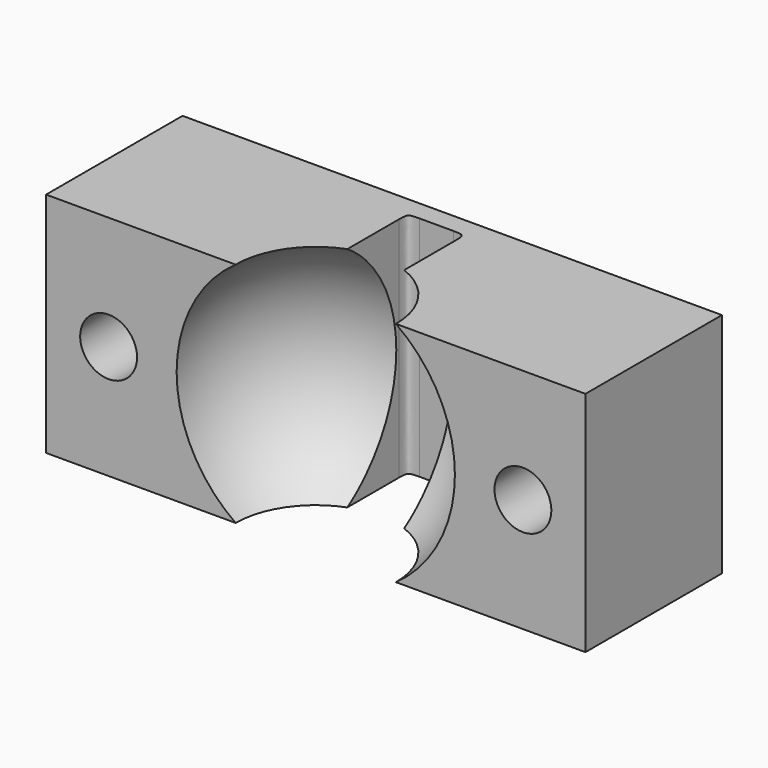
from build123d import *

# Parameters (mm, degrees)
F0_W        = 47.4317967892
F0_H        = 20
F0_R        = 4.5
F1_DEPTH    = 15
F2_R        = 7.05
F3_DEPTH    = 25
F7_DEPTH    = 13.25
F8_T1_DEPTH = 20
F0_R_2      = 2.5
F9_DEPTH    = 15


# Not quite as in the source:
# - a fillet or chamfer that OpenCascade refuses, or shapes differently, is made with other operations: its cross-section is extruded or revolved along the edge and cut away or added


with BuildPart() as f1:
    # F0 (on Front) → F1 (new body)
    with BuildSketch(Plane.XZ):
        Rectangle(F0_W, F0_H)
        with Locations((-18.2158983946, 0)):
            Circle(F0_R, mode=Mode.SUBTRACT)
        with Locations((18.2158983946, 0)):
            Circle(F0_R, mode=Mode.SUBTRACT)
    extrude(amount=F1_DEPTH)

    # F2 (on face) → F3 (cut)
    with BuildSketch(Plane.XY.offset(10)):
        with Locations((0, -15)):
            Circle(F2_R)
    extrude(amount=-F3_DEPTH, mode=Mode.SUBTRACT)

    # F4 (on face) → F5 (revolve, cut)
    with BuildSketch(Plane.XZ.offset(15)):
        with BuildLine():
            Line((-7.05, -10), (-7.05, 10))
            ThreePointArc((-7.05, 10), (-12.2352972992, 0), (-7.05, -10))
        make_face()
    revolve(axis=Axis((0, -15, 0.0368109904), (0, 0, -1)), mode=Mode.SUBTRACT)

    # F6 (on face) → F7 (cut)
    with BuildSketch(Plane.XZ.offset(15)):
        Polygon((2.5, -10.0813228637), (2.5, 10), (0, 10), (-2.5, 10), (-2.5, -10.0813228637), (0, -10.0813228637), align=None)
    extrude(amount=-F7_DEPTH, mode=Mode.SUBTRACT)

    # F8: fillet of radius 1 on 2 edges, made by hand

    # F8_s2 → F8_t1 (join)
    with BuildSketch(Plane.XY.offset(-10)):
        with BuildLine():
            add(Edge.make_bspline(
                [(1.5, -1.75), (2.5, -1.75), (2.5, -2.75)],
                knots=[0, 0, 0, 1, 1, 1], degree=2, weights=[1, 2.3333333333, 1]))
            Line((2.5, -2.75), (2.5, -1.75))
            Line((2.5, -1.75), (1.5, -1.75))
        make_face()
        with BuildLine():
            add(Edge.make_bspline(
                [(-2.5, -2.75), (-2.5, -1.75), (-1.5, -1.75)],
                knots=[0, 0, 0, 1, 1, 1], degree=2, weights=[1, 2.3333333333, 1]))
            Line((-1.5, -1.75), (-2.5, -1.75))
            Line((-2.5, -1.75), (-2.5, -2.75))
        make_face()
    extrude(amount=F8_T1_DEPTH)

    # F0 (on Front) → F9 (join)
    with BuildSketch(Plane.XZ):
        with Locations((-18.2158983946, 0)):
            Circle(F0_R)
        with Locations((-18.2158983946, 0)):
            Circle(F0_R_2, mode=Mode.SUBTRACT)
        with Locations((18.2158983946, 0)):
            Circle(F0_R)
        with Locations((18.2158983946, 0)):
            Circle(F0_R_2, mode=Mode.SUBTRACT)
    extrude(amount=F9_DEPTH)


solid = f1.part
